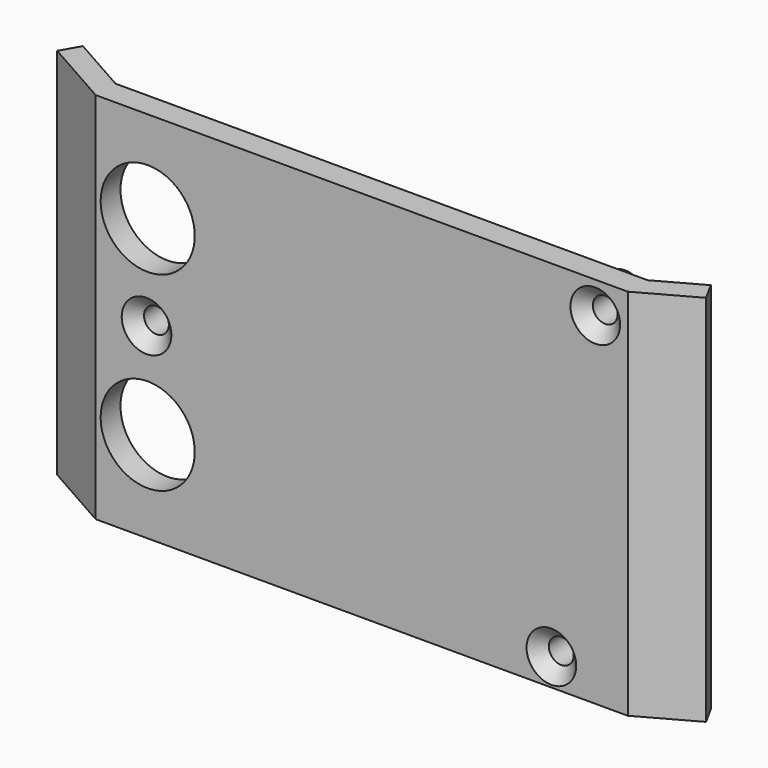
from build123d import *

# Parameters (mm, degrees)
F0_W            = 42.7
F0_H            = 30.1
F0_R            = 2
F1_DEPTH        = 2
F2_DEPTH        = 3
F3_DEPTH        = 0.1
F4_DEPTH        = 0.1
F6_W            = 1.7407113919
F6_H            = 30.1
F7_DEPTH        = 6.5
F9_W            = 1.7492394143
F9_H            = 30.1
F10_DEPTH       = 5
F11_D           = 2
F11_CSINK_D     = 4
F11_CSINK_ANGLE = 90
F12_D           = 7.59


# Not quite as in the source:
# - a feature names something its author has since deleted; it is built from what else it names


with BuildPart() as f1:
    # F0 (on Front) → F1 (new body)
    with BuildSketch(Plane.XZ):
        Rectangle(F0_W, F0_H)
        with Locations((-17.35, 0)):
            Circle(F0_R, mode=Mode.SUBTRACT)
        with Locations((15.29, -12.86)):
            Circle(F0_R, mode=Mode.SUBTRACT)
        with Locations((18.83, 12.5)):
            Circle(F0_R, mode=Mode.SUBTRACT)
        with Locations((18.83, 12.5)):
            Circle(F0_R)
        with Locations((-17.35, 0)):
            Circle(F0_R)
        with Locations((15.29, -12.86)):
            Circle(F0_R)
    extrude(amount=-F1_DEPTH)

    # F0 (on Front) → F2 (join)
    with BuildSketch(Plane.XZ):
        with Locations((18.83, 12.5)):
            Circle(F0_R)
        with Locations((15.29, -12.86)):
            Circle(F0_R)
        with Locations((-17.35, 0)):
            Circle(F0_R)
    extrude(amount=-F2_DEPTH)

    # F3 (add): a face of the model
    f3_faces = [f1.faces().sort_by_distance(p)[0] for p in [
        (-21.35, 1, 0),
    ]]
    extrude(f3_faces, amount=F3_DEPTH)

    # F4 (add): a face of the model
    f4_faces = [f1.faces().sort_by_distance(p)[0] for p in [
        (21.35, 1, 0),
    ]]
    extrude(f4_faces, amount=F4_DEPTH)

    # F6 (on face) → F7 (join)
    with BuildSketch(Plane(origin=(-16.2487833534, 9.1931193, 0), x_dir=(0.4924235601, 0.8703556959, 0), z_dir=(0.8703556959, -0.4924235601, 0))):
        with Locations((-9.6921296683, 0)):
            Rectangle(F6_W, F6_H)
    extrude(amount=-F7_DEPTH)

    # F9 (on face) → F10 (join)
    with BuildSketch(Plane(origin=(16.4083841089, 9.0953158313, 0), x_dir=(0.4848096202, -0.8746197071, 0), z_dir=(-0.8746197071, -0.4848096202, 0))):
        with Locations((9.5245466471, 0)):
            Rectangle(F9_W, F9_H)
    extrude(amount=-F10_DEPTH)

    # F11 (through all)
    with Locations(Plane.XZ):
        with Locations((-17.35, 0), (18.83, 12.5), (15.29, -12.86)):
            CounterSinkHole(F11_D / 2, F11_CSINK_D / 2, counter_sink_angle=F11_CSINK_ANGLE)

    # F12 (through all)
    with Locations(Plane.XZ):
        with Locations((-17.255, 7.655), (-17.255, -7.695)):
            Hole(F12_D / 2)


solid = f1.part
